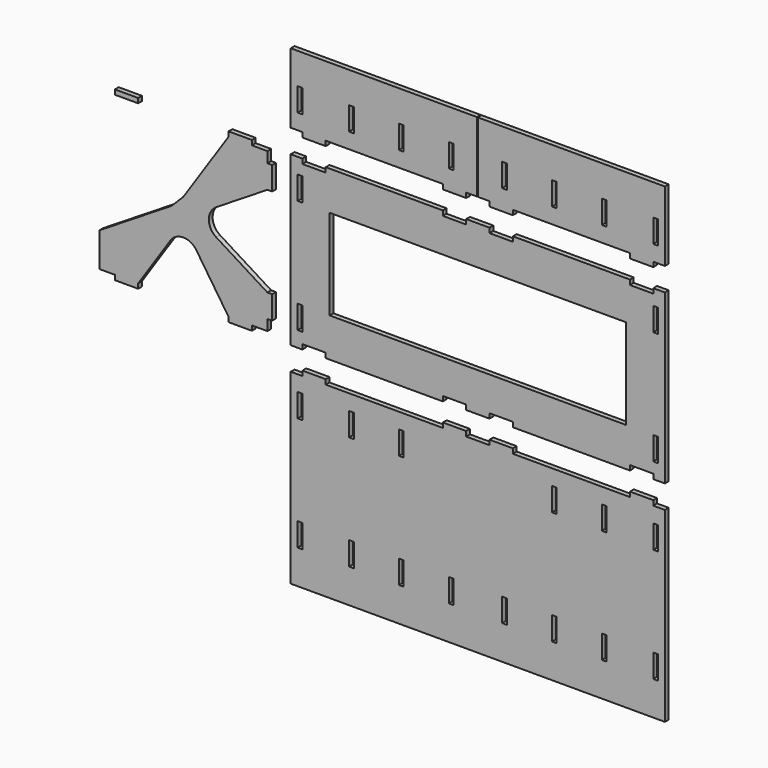
from build123d import *

# Parameters (mm, degrees)
F0_W     = 15.494
F0_H     = 76.2
F0_W_2   = 968.375
F0_H_2   = 295.275
F1_DEPTH = 15.494
F0_W_3   = 76.2
F0_H_3   = 15.748
F0_H_4   = 15.494
F2_R     = 50.8


# Not quite as in the source:
# - a feature names something its author has since deleted; it is built from what else it names


with BuildPart() as f1:
    # F0 (on Front) → F1 (new body)
    with BuildSketch(Plane.XZ):
        Polygon((611.1875, -274.6375), (611.1875, 274.6375), (573.0875, 274.6375), (573.0875, 258.8895), (496.8875, 258.8895), (496.8875, 274.6375), (114.3, 274.6375), (114.3, 258.8895), (38.1, 258.8895), (38.1, 274.6375), (-38.1, 274.6375), (-38.1, 258.8895), (-114.3, 258.8895), (-114.3, 274.6375), (-496.8875, 274.6375), (-496.8875, 258.8895), (-573.0875, 258.8895), (-573.0875, 274.6375), (-611.1875, 274.6375), (-611.1875, -274.6375), (-573.0875, -274.6375), (-573.0875, -258.8895), (-496.8875, -258.8895), (-496.8875, -274.6375), (-114.3, -274.6375), (-114.3, -258.8895), (-38.1, -258.8895), (-38.1, -274.6375), (38.1, -274.6375), (38.1, -258.8895), (114.3, -258.8895), (114.3, -274.6375), (496.8875, -274.6375), (496.8875, -258.8895), (573.0875, -258.8895), (573.0875, -274.6375), align=None)
        with Locations((-580.8345, -185.7375)):
            Rectangle(F0_W, F0_H, mode=Mode.SUBTRACT)
        with Locations((580.8345, -185.7375)):
            Rectangle(F0_W, F0_H, mode=Mode.SUBTRACT)
        with Locations((-580.8345, 185.7375)):
            Rectangle(F0_W, F0_H, mode=Mode.SUBTRACT)
        Rectangle(F0_W_2, F0_H_2, mode=Mode.SUBTRACT)
        with Locations((580.8345, 185.7375)):
            Rectangle(F0_W, F0_H, mode=Mode.SUBTRACT)
    extrude(amount=F1_DEPTH)


with BuildPart() as f1b:
    # F0 (on Front) → F1, piece 2 (new body)
    with BuildSketch(Plane.XZ):
        Polygon((-611.1875, 579.4375), (-611.1875, 350.8375), (-573.0875, 350.8375), (-496.8875, 350.8375), (-114.3, 350.8375), (-38.1, 350.8375), (-3.175, 350.8375), (-3.175, 579.4375), align=None)
        with Locations((-580.8345, 439.7375)):
            Rectangle(F0_W, F0_H, mode=Mode.SUBTRACT)
        with Locations((-412.9405, 439.7375)):
            Rectangle(F0_W, F0_H, mode=Mode.SUBTRACT)
        with Locations((-250.03125, 439.7375)):
            Rectangle(F0_W, F0_H, mode=Mode.SUBTRACT)
        with Locations((-87.122, 439.7375)):
            Rectangle(F0_W, F0_H, mode=Mode.SUBTRACT)
        with Locations((-534.9875, 342.9635)):
            Rectangle(F0_W_3, F0_H_3)
        with Locations((-76.2, 342.9635)):
            Rectangle(F0_W_3, F0_H_3)
    extrude(amount=F1_DEPTH)


with BuildPart() as f1c:
    # F0 (on Front) → F1, piece 3 (new body)
    with BuildSketch(Plane.XZ):
        Polygon((573.0875, 350.8375), (611.1875, 350.8375), (611.1875, 579.4375), (0, 579.4375), (0, 350.8375), (38.1, 350.8375), (114.3, 350.8375), (496.8875, 350.8375), align=None)
        with Locations((87.122, 439.7375)):
            Rectangle(F0_W, F0_H, mode=Mode.SUBTRACT)
        with Locations((250.03125, 439.7375)):
            Rectangle(F0_W, F0_H, mode=Mode.SUBTRACT)
        with Locations((412.9405, 439.7375)):
            Rectangle(F0_W, F0_H, mode=Mode.SUBTRACT)
        with Locations((580.8345, 439.7375)):
            Rectangle(F0_W, F0_H, mode=Mode.SUBTRACT)
        with Locations((534.9875, 342.9635)):
            Rectangle(F0_W_3, F0_H_3)
        with Locations((76.2, 342.9635)):
            Rectangle(F0_W_3, F0_H_3)
    extrude(amount=F1_DEPTH)


with BuildPart() as f1d:
    # F0 (on Front) → F1, piece 4 (new body)
    with BuildSketch(Plane.XZ):
        Polygon((-687.3875, 223.8375), (-687.3875, 258.8895), (-738.1875, 258.8895), (-814.3875, 258.8895), (-962.025, 38.1), (-1000.125, 0), (-1236.6625, -147.6375), (-1236.6625, -258.8895), (-1185.8625, -258.8895), (-1109.6625, -258.8895), (-962.025, -38.1), (-814.3875, -258.8895), (-738.1875, -258.8895), (-687.3875, -258.8895), (-687.3875, -223.8375), (-687.3875, -147.6375), (-923.925, 0), (-687.3875, 147.6375), align=None)
        with Locations((-776.2875, 266.6365)):
            Rectangle(F0_W_3, F0_H_4)
        with Locations((-679.6405, 185.7375)):
            Rectangle(F0_W, F0_H)
        with Locations((-679.6405, -185.7375)):
            Rectangle(F0_W, F0_H)
        with Locations((-776.2875, -266.6365)):
            Rectangle(F0_W_3, F0_H_4)
        with Locations((-1147.7625, -266.6365)):
            Rectangle(F0_W_3, F0_H_4)
    extrude(amount=F1_DEPTH)

    # F2
    f2_edges = [f1d.edges().sort_by_distance(p)[0] for p in [
        (-1000.125, -7.747, 0),
        (-962.025, -7.747, 38.1),
        (-923.925, -7.747, 0),
        (-962.025, -7.747, -38.1),
    ]]
    fillet(f2_edges, radius=F2_R)


with BuildPart() as f1e:
    # F0 (on Front) → F1, piece 5 (new body)
    with BuildSketch(Plane.XZ):
        with Locations((-1147.7625, 266.6365)):
            Rectangle(F0_W_3, F0_H_4)
    extrude(amount=F1_DEPTH)


with BuildPart() as f1f:
    # F0 (on Front) → F1, piece 6 (new body)
    with BuildSketch(Plane.XZ):
        with Locations((-76.2, -342.9635)):
            Rectangle(F0_W_3, F0_H_3)
        Polygon((-38.1, -350.8375), (-114.3, -350.8375), (-496.8875, -350.8375), (-573.0875, -350.8375), (-611.1875, -350.8375), (-611.1875, -960.4375), (611.1875, -960.4375), (611.1875, -350.8375), (573.0875, -350.8375), (496.8875, -350.8375), (114.3, -350.8375), (38.1, -350.8375), align=None)
        with Locations((-580.8345, -811.2125)):
            Rectangle(F0_W, F0_H, mode=Mode.SUBTRACT)
        with Locations((-412.9405, -811.2125)):
            Rectangle(F0_W, F0_H, mode=Mode.SUBTRACT)
        with Locations((-580.8345, -439.7375)):
            Rectangle(F0_W, F0_H, mode=Mode.SUBTRACT)
        with Locations((-412.9405, -439.7375)):
            Rectangle(F0_W, F0_H, mode=Mode.SUBTRACT)
        with Locations((-250.03125, -811.2125)):
            Rectangle(F0_W, F0_H, mode=Mode.SUBTRACT)
        with Locations((-87.122, -811.2125)):
            Rectangle(F0_W, F0_H, mode=Mode.SUBTRACT)
        with Locations((87.122, -811.2125)):
            Rectangle(F0_W, F0_H, mode=Mode.SUBTRACT)
        with Locations((250.03125, -811.2125)):
            Rectangle(F0_W, F0_H, mode=Mode.SUBTRACT)
        with Locations((412.9405, -811.2125)):
            Rectangle(F0_W, F0_H, mode=Mode.SUBTRACT)
        with Locations((580.8345, -811.2125)):
            Rectangle(F0_W, F0_H, mode=Mode.SUBTRACT)
        with Locations((-250.03125, -439.7375)):
            Rectangle(F0_W, F0_H, mode=Mode.SUBTRACT)
        with Locations((250.03125, -439.7375)):
            Rectangle(F0_W, F0_H, mode=Mode.SUBTRACT)
        with Locations((412.9405, -439.7375)):
            Rectangle(F0_W, F0_H, mode=Mode.SUBTRACT)
        with Locations((580.8345, -439.7375)):
            Rectangle(F0_W, F0_H, mode=Mode.SUBTRACT)
        with Locations((-534.9875, -342.9635)):
            Rectangle(F0_W_3, F0_H_3)
        with Locations((76.2, -342.9635)):
            Rectangle(F0_W_3, F0_H_3)
        with Locations((534.9875, -342.9635)):
            Rectangle(F0_W_3, F0_H_3)
    extrude(amount=F1_DEPTH)


solid = Compound([f1.part, f1b.part, f1c.part, f1d.part, f1e.part, f1f.part])
